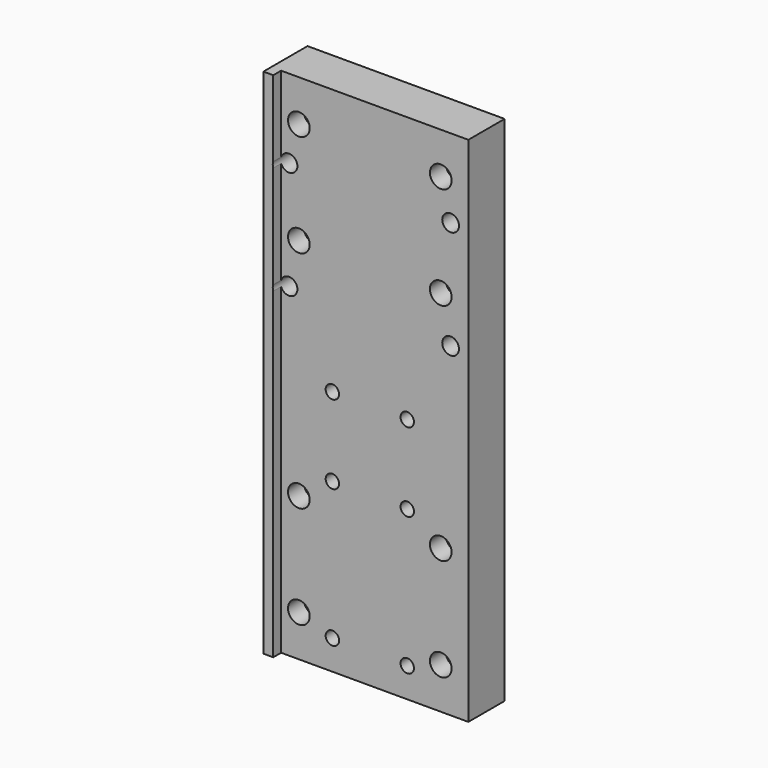
from build123d import *

# Parameters (mm, degrees)
F0_W           = 5
F0_H           = 260
F1_DEPTH       = 28
F0_W_2         = 95
F2_DEPTH       = 23
F3_D           = 8.5
F4_D           = 6.8
F5_D           = 11
F5_CBORE_D     = 19
F5_CBORE_DEPTH = 13


# Not quite as in the source:
# - a feature names something its author has since deleted; it is built from what else it names


with BuildPart() as f1:
    # F0 (on Front) → F1 (new body)
    with BuildSketch(Plane.XZ):
        with Locations((-47.5, 0)):
            Rectangle(F0_W, F0_H)
    extrude(amount=F1_DEPTH)

    # F0 (on Front) → F2 (join)
    with BuildSketch(Plane.XZ):
        with Locations((2.5, 0)):
            Rectangle(F0_W_2, F0_H)
    extrude(amount=F2_DEPTH)

    # F3 (through all)
    with Locations(Plane(origin=(0, 0, 0), x_dir=(1, 0, 0), z_dir=(0, 1, 0))):
        with Locations((41, -90), (-41, -90), (41, -35), (-41, -35)):
            Hole(F3_D / 2)

    # F4 (through all)
    with Locations(Plane(origin=(0, 0, 0), x_dir=(1, 0, 0), z_dir=(0, 1, 0))):
        with Locations((19, 5), (-19, 5), (19, 45), (-19, 45), (19, 115), (-19, 115)):
            Hole(F4_D / 2)

    # F5 (through all)
    with Locations(Plane(origin=(0, 0, 0), x_dir=(1, 0, 0), z_dir=(0, 1, 0))):
        with Locations((36, -109), (-36, -109), (36, -57), (-36, -57), (36, 57), (-36, 57), (-36, 109), (36, 109)):
            CounterBoreHole(F5_D / 2, F5_CBORE_D / 2, F5_CBORE_DEPTH)


solid = f1.part
